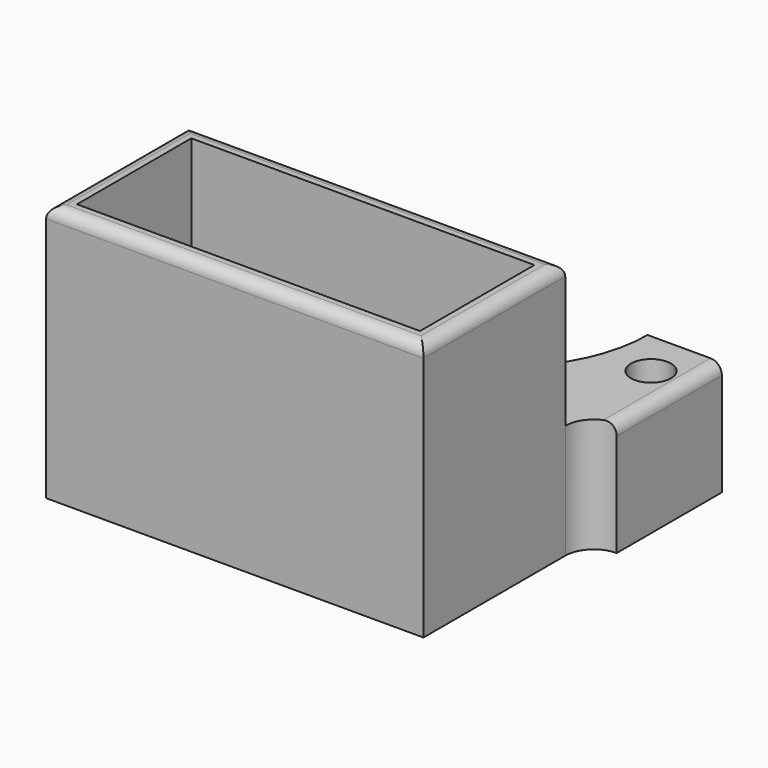
from build123d import *

# Parameters (mm, degrees)
F0_W     = 60
F0_H     = 25
F1_DEPTH = 45
F0_R     = 3.5
F2_DEPTH = 20
F4_R     = 2
F4_2_R   = 2


# Not quite as in the source:
# - a feature of the source that left no trace in its solid (it failed there, or was rolled back) is left out


with BuildPart() as f1:
    # F0 (on Top) → F1 (new body)
    with BuildSketch(Plane.XY):
        Polygon((-33, -15.5), (33, -15.5), (33, 15.5), (0, 15.5), (-33, 15.5), align=None)
        Rectangle(F0_W, F0_H, mode=Mode.SUBTRACT)
    extrude(amount=F1_DEPTH)

    # F4#2
    f4_2_edges = [f1.edges().sort_by_distance(p)[0] for p in [
        (0, -15.5, 45),
        (33, 0, 45),
        (0, 15.5, 45),
        (-33, 0, 45),
    ]]
    fillet(f4_2_edges, radius=F4_2_R)


with BuildPart() as f2:
    # F0 (on Top) → F2 (new body)
    with BuildSketch(Plane.XY):
        with BuildLine():
            Line((0, 15.5), (33, 15.5))
            ThreePointArc((33, 15.5), (34.4644660941, 19.0355339059), (38, 20.5))
            Line((38, 20.5), (38, 43.5))
            Line((38, 43.5), (28, 43.5))
            ThreePointArc((28, 43.5), (19.7989898732, 23.7010101268), (0, 15.5))
        make_face()
        with Locations((32, 35.5)):
            Circle(F0_R, mode=Mode.SUBTRACT)
        with BuildLine():
            ThreePointArc((-28, 43.5), (-19.7989898732, 23.7010101268), (0, 15.5))
            ThreePointArc((0, 15.5), (19.7989898732, 23.7010101268), (28, 43.5))
            Line((28, 43.5), (25, 43.5))
            ThreePointArc((25, 43.5), (0, 18.5), (-25, 43.5))
            Line((-25, 43.5), (-28, 43.5))
        make_face()
        with BuildLine():
            ThreePointArc((-38, 20.5), (-34.4644660941, 19.0355339059), (-33, 15.5))
            Line((-33, 15.5), (0, 15.5))
            ThreePointArc((0, 15.5), (-19.7989898732, 23.7010101268), (-28, 43.5))
            Line((-28, 43.5), (-38, 43.5))
            Line((-38, 43.5), (-38, 20.5))
        make_face()
        with Locations((-32, 35.5)):
            Circle(F0_R, mode=Mode.SUBTRACT)
    extrude(amount=F2_DEPTH)

    # F4
    f4_edges = [f2.edges().sort_by_distance(p)[0] for p in [
        (-38, 20.5, 10),
        (38, 32, 20),
        (-38, 32, 20),
        (-34.464466, 19.035534, 20),
    ]]
    fillet(f4_edges, radius=F4_R)


solid = Compound([f1.part, f2.part])
